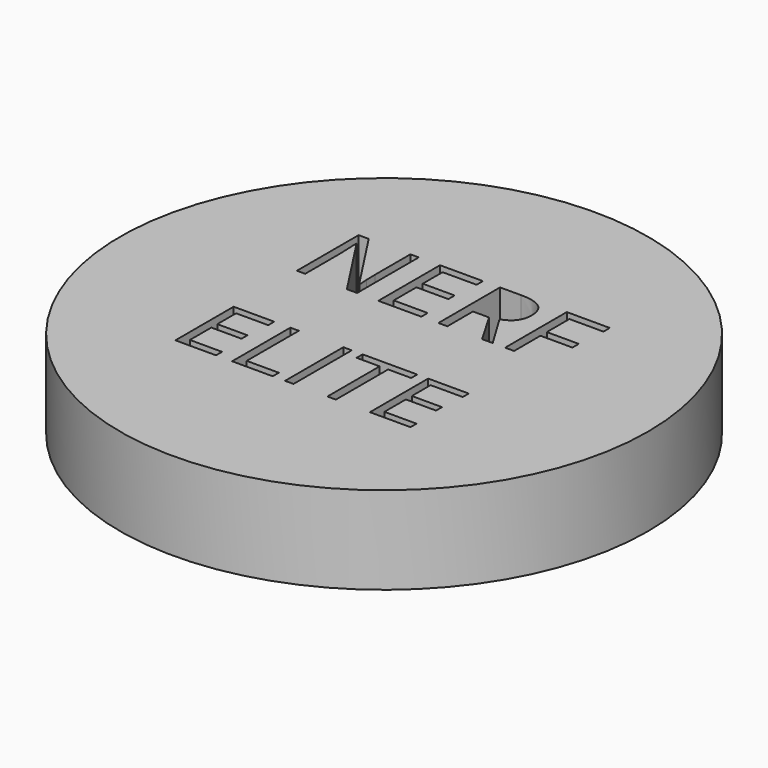
from build123d import *

# Parameters (mm, degrees)
F0_R     = 76.4498287505
F0_W     = 2.4511385491
F0_H     = 21.0908701144
F1_DEPTH = 25.4


# Not quite as in the source:
# - a feature names something its author has since deleted; it is built from what else it names


with BuildPart() as f1:
    # F0 (on Top) → F1 (new body)
    with BuildSketch(Plane.XY):
        Circle(F0_R)
        with BuildLine():
            Line((-18.3724183589, -37.9301533103), (-18.3724183589, -42.5397194922))
            ThreePointArc((-18.3724183589, -42.5397194922), (-20.6772014499, -40.2349364012), (-18.3724183589, -37.9301533103))
        make_face(mode=Mode.SUBTRACT)
        Polygon((-23.2161222044, -29.6504020767), (-23.2161222044, -31.8430401385), (-34.9732782957, -31.8430401385), (-34.9732782957, -10.7521700241), (-23.2161222044, -10.7521700241), (-23.2161222044, -12.9309598455), (-32.5221397466, -12.9309598455), (-32.5221397466, -19.725829797), (-23.7792839802, -19.725829797), (-23.7792839802, -21.890771378), (-32.5221397466, -21.890771378), (-32.5221397466, -29.6504020767), align=None, mode=Mode.SUBTRACT)
        Polygon((-6.7874930214, -31.8430401385), (-18.5446491127, -31.8430401385), (-18.5446491127, -10.7521700241), (-16.0935105636, -10.7521700241), (-16.0935105636, -29.6227055959), (-6.7874930214, -29.6227055959), align=None, mode=Mode.SUBTRACT)
        with Locations((-1.984461646, -21.2976050813)):
            Rectangle(F0_W, F0_H, mode=Mode.SUBTRACT)
        Polygon((11.5152646944, -12.9309598455), (11.5152646944, -31.8430401385), (9.0641261454, -31.8430401385), (9.0641261454, -12.9309598455), (2.3846581971, -12.9309598455), (2.3846581971, -10.7521700241), (18.1947326427, -10.7521700241), (18.1947326427, -12.9309598455), align=None, mode=Mode.SUBTRACT)
        Polygon((33.1277518635, -29.6504020767), (33.1277518635, -31.8430401385), (21.3705957722, -31.8430401385), (21.3705957722, -10.7521700241), (33.1277518635, -10.7521700241), (33.1277518635, -12.9309598455), (23.8217343212, -12.9309598455), (23.8217343212, -19.725829797), (32.5645900876, -19.725829797), (32.5645900876, -21.890771378), (23.8217343212, -21.890771378), (23.8217343212, -29.6504020767), align=None, mode=Mode.SUBTRACT)
        with BuildLine():
            Line((-17.3598606786, 34.2694889666), (-17.3598606786, 11.9390692562))
            Line((-17.3598606786, 11.9390692562), (-20.321610371, 11.9390692562))
            Line((-20.321610371, 11.9390692562), (-32.5253875688, 30.677267805))
            Line((-32.5253875688, 30.677267805), (-32.647571962, 30.677267805))
            add(Edge.make_bspline(
                [(-32.647571962, 30.677267805), (-32.4032031755, 27.3782891873), (-32.4032031755, 24.631584027)],
                knots=[0, 0, 0, 1, 1, 1], degree=2))
            Line((-32.4032031755, 24.631584027), (-32.4032031755, 11.9390692562))
            Line((-32.4032031755, 11.9390692562), (-34.8029046589, 11.9390692562))
            Line((-34.8029046589, 11.9390692562), (-34.8029046589, 34.2694889666))
            Line((-34.8029046589, 34.2694889666), (-31.8704792209, 34.2694889666))
            Line((-31.8704792209, 34.2694889666), (-19.6960262775, 15.6046010537))
            Line((-19.6960262775, 15.6046010537), (-19.5738418843, 15.6046010537))
            add(Edge.make_bspline(
                [(-19.5738418843, 15.6046010537), (-19.6031661386, 16.015140615), (-19.7106884047, 18.2535586993)],
                knots=[0, 0, 0, 1, 1, 1], degree=2))
            add(Edge.make_bspline(
                [(-19.7106884047, 18.2535586993), (-19.8182106708, 20.4919767837), (-19.7888864164, 21.4547898025)],
                knots=[0, 0, 0, 1, 1, 1], degree=2))
            Line((-19.7888864164, 21.4547898025), (-19.7888864164, 34.2694889666))
            Line((-19.7888864164, 34.2694889666), (-17.3598606786, 34.2694889666))
        make_face(mode=Mode.SUBTRACT)
        Polygon((1.2268292226, 14.2605727279), (1.2268292226, 11.9390692562), (-11.2213167617, 11.9390692562), (-11.2213167617, 34.2694889666), (1.2268292226, 34.2694889666), (1.2268292226, 31.962647622), (-8.6261202491, 31.962647622), (-8.6261202491, 24.7684305474), (0.6305693836, 24.7684305474), (0.6305693836, 22.4762513301), (-8.6261202491, 22.4762513301), (-8.6261202491, 14.2605727279), align=None, mode=Mode.SUBTRACT)
        with BuildLine():
            Line((13.4306064204, 21.2250831432), (8.768049974, 21.2250831432))
            Line((8.768049974, 21.2250831432), (8.768049974, 11.9390692562))
            Line((8.768049974, 11.9390692562), (6.1728534614, 11.9390692562))
            Line((6.1728534614, 11.9390692562), (6.1728534614, 34.2694889666))
            Line((6.1728534614, 34.2694889666), (12.2967352511, 34.2694889666))
            add(Edge.make_bspline(
                [(12.2967352511, 34.2694889666), (16.40701824, 34.2694889666), (18.3692995956, 32.6957539815)],
                knots=[0, 0, 0, 1, 1, 1], degree=2))
            add(Edge.make_bspline(
                [(18.3692995956, 32.6957539815), (20.3315809512, 31.1220189964), (20.3315809512, 27.9598868991)],
                knots=[0, 0, 0, 1, 1, 1], degree=2))
            add(Edge.make_bspline(
                [(20.3315809512, 27.9598868991), (20.3315809512, 23.5319244877), (15.8400826553, 21.9728516299)],
                knots=[0, 0, 0, 1, 1, 1], degree=2))
            Line((15.8400826553, 21.9728516299), (21.9053159362, 11.9390692562))
            Line((21.9053159362, 11.9390692562), (18.8360439778, 11.9390692562))
            Line((18.8360439778, 11.9390692562), (13.4306064204, 21.2250831432))
        make_face(mode=Mode.SUBTRACT)
        Polygon((28.1025083619, 21.4841140569), (28.1025083619, 11.9390692562), (25.5073118492, 11.9390692562), (25.5073118492, 34.2694889666), (37.9554578336, 34.2694889666), (37.9554578336, 31.962647622), (28.1025083619, 31.962647622), (28.1025083619, 23.7909554014), (37.3591979945, 23.7909554014), (37.3591979945, 21.4841140569), align=None, mode=Mode.SUBTRACT)
        with BuildLine():
            ThreePointArc((-18.3724183589, -37.9301533103), (-20.6772014499, -40.2349364012), (-18.3724183589, -42.5397194922))
            Line((-18.3724183589, -42.5397194922), (-18.3724183589, -37.9301533103))
        make_face()
    extrude(amount=F1_DEPTH)


solid = f1.part
